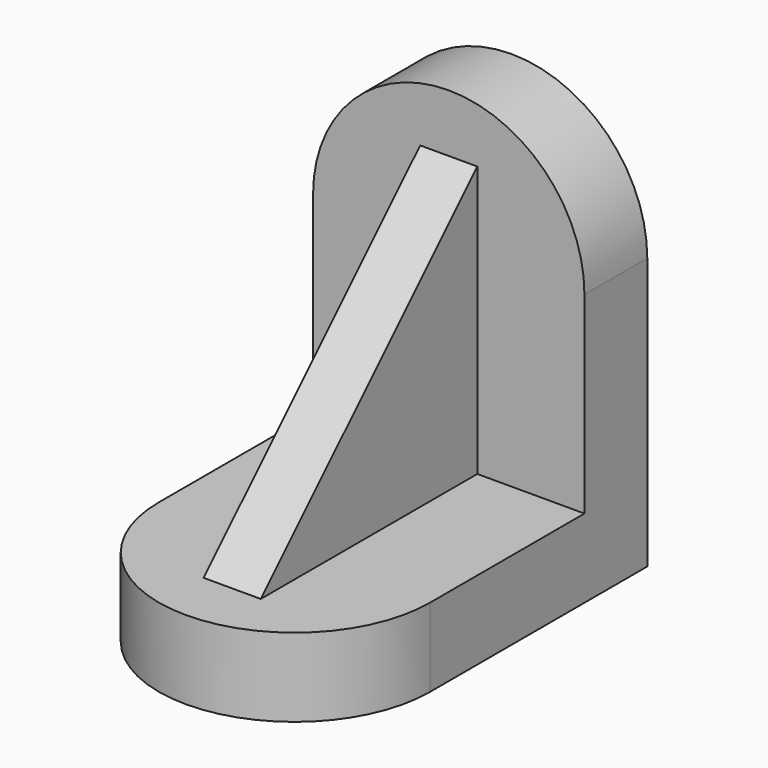
from build123d import *

# Parameters (mm, degrees)
F1_DEPTH    = 11
F3_DEPTH    = 11
F5_W        = 8
F5_H        = 38
F6_DEPTH    = 38
F7_T4_DEPTH = 203.4479070854


# Not quite as in the source:
# - a fillet or chamfer that OpenCascade refuses, or shapes differently, is made with other operations: its cross-section is extruded or revolved along the edge and cut away or added


with BuildPart() as f1:
    # F0 (on Front) → F1 (new body)
    with BuildSketch(Plane.XZ):
        with BuildLine():
            Line((0, 38), (0, 0))
            Line((0, 0), (38, 0))
            Line((38, 0), (38, 38))
            ThreePointArc((38, 38), (19, 57), (0, 38))
        make_face()
    extrude(amount=F1_DEPTH)

    # F2 (on Top) → F3 (join)
    with BuildSketch(Plane.XY):
        with BuildLine():
            Line((38, 0), (0, 0))
            Line((0, 0), (0, -38))
            ThreePointArc((0, -38), (19, -57), (38, -38))
            Line((38, -38), (38, 0))
        make_face()
    extrude(amount=F3_DEPTH)

    # F5 (on offset) → F6 (join)
    with BuildSketch(Plane.XZ.offset(11)):
        with Locations((19, 29.9000790417)):
            Rectangle(F5_W, F5_H)
    extrude(amount=F6_DEPTH)

    # F7: chamfer of 38 on 1 edges, made by hand


with BuildPart() as f7_tool2:
    # F7_s3 → F7_t4 (new body)
    with BuildSketch(Plane.YZ.offset(120.7239535427)):
        Polygon((-11, 48.9000790417), (-49, 10.9000790417), (-49, 48.9000790417), align=None)
    extrude(amount=-F7_T4_DEPTH)

    split(bisect_by=Plane.XZ.offset(11), keep=Keep.TOP)

    split(bisect_by=Plane.XY.offset(11), keep=Keep.TOP)


with BuildPart() as f1_1:
    add(f1.part)

    # F7_t1: cut F7_tool2
    add(f7_tool2.part, mode=Mode.SUBTRACT)


solid = f1_1.part
